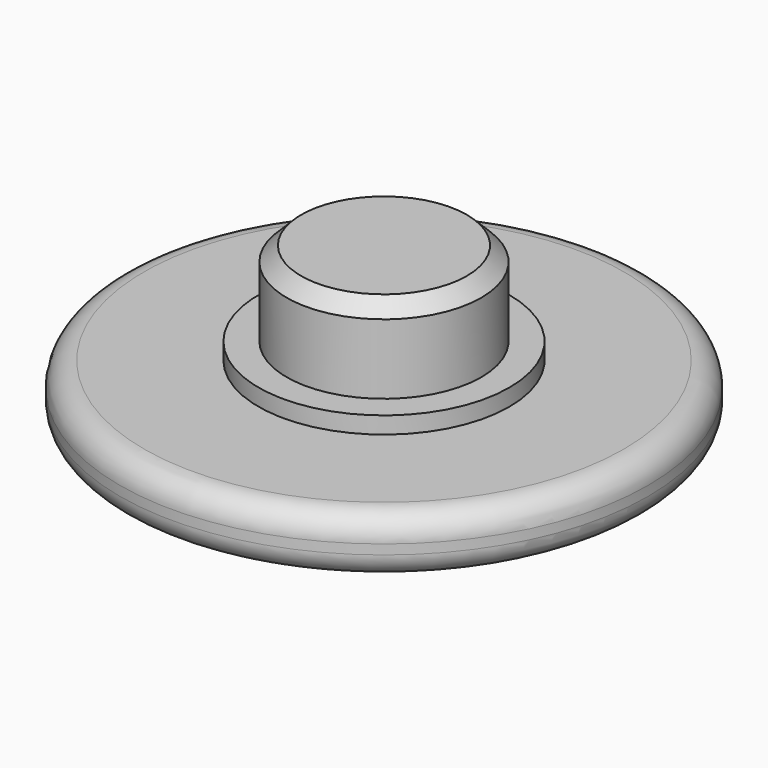
from build123d import *

# Parameters (mm, degrees)
F0_R     = 10.95
F1_DEPTH = 2.4
F2_R     = 4.035
F3_DEPTH = 4.2
F4_R     = 1
F5_R     = 5.2
F5_R_2   = 4.035
F6_DEPTH = 0.7
F7_R     = 1
F8_R     = 8
F9_DEPTH = 1
F11_SIZE = 0.6
F12_R    = 6


# Not quite as in the source:
# - a fillet or chamfer that OpenCascade refuses, or shapes differently, is made with other operations: its cross-section is extruded or revolved along the edge and cut away or added


with BuildPart() as f1:
    # F0 (on Top) → F1 (new body)
    with BuildSketch(Plane.XY):
        Circle(F0_R)
    extrude(amount=F1_DEPTH)

    # F2 (on face) → F3 (join)
    with BuildSketch(Plane.XY.offset(2.4)):
        Circle(F2_R)
    extrude(amount=F3_DEPTH)

    # F4
    f4_edges = [f1.edges().sort_by_distance(p)[0] for p in [
        (-10.95, 0, 2.4),
    ]]
    fillet(f4_edges, radius=F4_R)

    # F5 (on face) → F6 (join)
    with BuildSketch(Plane.XY.offset(2.4)):
        Circle(F5_R)
        Circle(F5_R_2, mode=Mode.SUBTRACT)
    extrude(amount=F6_DEPTH)

    # F7
    f7_edges = [f1.edges().sort_by_distance(p)[0] for p in [
        (-10.95, 0, 0),
    ]]
    fillet(f7_edges, radius=F7_R)

    # F8 (on face) → F9 (cut)
    with BuildSketch(Plane(origin=(0, 0, 0), x_dir=(1, 0, 0), z_dir=(0, 0, -1))):
        Circle(F8_R)
    extrude(amount=-F9_DEPTH, mode=Mode.SUBTRACT)

    # F10: fillet of radius 11 on 1 edges, made by hand

    # F10_s1 → F10_t2 (revolve)
    with BuildSketch(Plane.XZ):
        with BuildLine():
            ThreePointArc((8, 0), (5.762632185, 0.7470926301), (3.417424305, 1))
            Line((3.417424305, 1), (8, 1))
            Line((8, 1), (8, 0))
        make_face()
    revolve(axis=Axis((0, 0, 1), (0, 0, -1)))

    # F11
    f11_edges = [f1.edges().sort_by_distance(p)[0] for p in [
        (-4.035, 0, 6.6),
    ]]
    chamfer(f11_edges, length=F11_SIZE)

    # F12
    f12_edges = [f1.edges().sort_by_distance(p)[0] for p in [
        (-8, 0, 0),
    ]]
    fillet(f12_edges, radius=F12_R)


solid = f1.part
